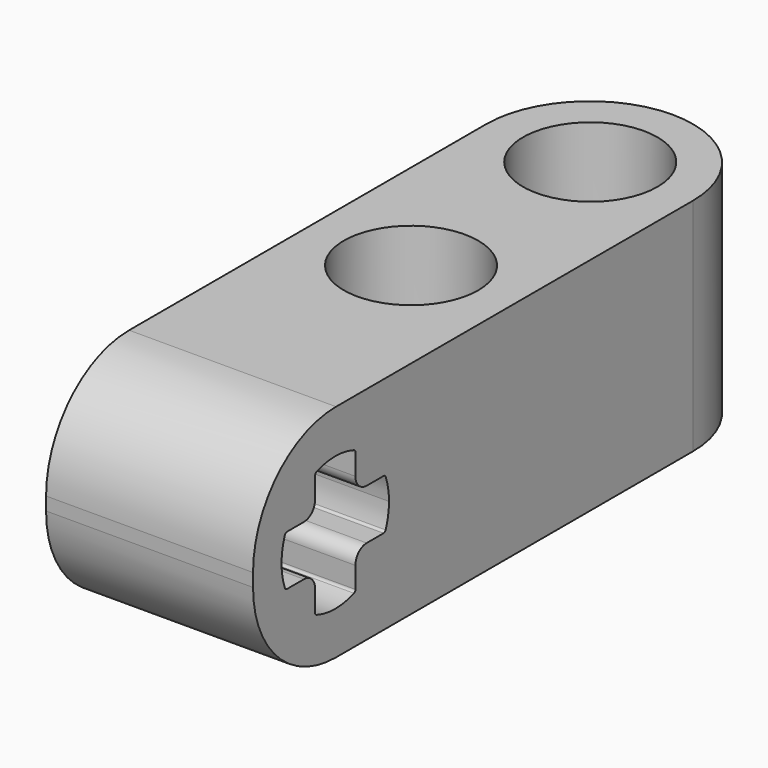
from build123d import *

# Parameters (mm, degrees)
F0_W        = 7.39
F0_H        = 23.34
F0_R        = 2.4
F1_DEPTH    = 7.88
F2_T1_DEPTH = 26.405
F4_DEPTH    = 7.391
F5_R        = 3.705


# Not quite as in the source:
# - a fillet or chamfer that OpenCascade refuses, or shapes differently, is made with other operations: its cross-section is extruded or revolved along the edge and cut away or added


with BuildPart() as f1:
    # F0 (on Top) → F1 (new body)
    with BuildSketch(Plane.XY):
        with Locations((-61.1013304442, -8.6294944299)):
            Rectangle(F0_W, F0_H)
        with Locations((-61.1013304442, -8.6294944299)):
            Circle(F0_R, mode=Mode.SUBTRACT)
        with Locations((-61.1013304442, -0.6294944299)):
            Circle(F0_R, mode=Mode.SUBTRACT)
    extrude(amount=F1_DEPTH)

    # F2: fillet of radius 3.705 on 2 edges, made by hand

    # F2_s2 → F2_t1 (cut)
    with BuildSketch(Plane.XY.offset(-9.2625)):
        with BuildLine():
            ThreePointArc((-61.0913304442, 3.0405055701), (-63.7111610685, 1.9553361944), (-64.7963304442, -0.6644944299))
            Line((-64.7963304442, -0.6644944299), (-64.7963304442, 3.0405055701))
            Line((-64.7963304442, 3.0405055701), (-61.0913304442, 3.0405055701))
        make_face()
        with BuildLine():
            ThreePointArc((-61.1113304442, 3.0405055701), (-58.4914998199, 1.9553361944), (-57.4063304442, -0.6644944299))
            Line((-57.4063304442, -0.6644944299), (-57.4063304442, 3.0405055701))
            Line((-57.4063304442, 3.0405055701), (-61.1113304442, 3.0405055701))
        make_face()
    extrude(amount=F2_T1_DEPTH, mode=Mode.SUBTRACT)

    # F3 (on face) → F4 (cut, through all)
    with BuildSketch(Plane.YZ.offset(-57.4063304442)):
        with BuildLine():
            Line((-15.7294944299, 5.34), (-15.7294944299, 6.0963858653))
            ThreePointArc((-15.7294944299, 6.0963858653), (-15.747402223, 6.1534898894), (-15.7947118212, 6.1901417725))
            ThreePointArc((-15.7947118212, 6.1901417725), (-16.6294944299, 6.34), (-17.4642770386, 6.1901417725))
            ThreePointArc((-17.4642770386, 6.1901417725), (-17.5115866368, 6.1534898894), (-17.5294944299, 6.0963858653))
            Line((-17.5294944299, 6.0963858653), (-17.5294944299, 5.34))
            ThreePointArc((-17.5294944299, 5.34), (-17.6759410393, 4.9864466094), (-18.0294944299, 4.84))
            Line((-18.0294944299, 4.84), (-18.7858802952, 4.84))
            ThreePointArc((-18.7858802952, 4.84), (-18.8429843193, 4.8220922069), (-18.8796362024, 4.7747826087))
            ThreePointArc((-18.8796362024, 4.7747826087), (-18.9917328021, 4.3640635248), (-19.0294944299, 3.94))
            ThreePointArc((-19.0294944299, 3.94), (-18.9917328021, 3.5159364752), (-18.8796362024, 3.1052173913))
            ThreePointArc((-18.8796362024, 3.1052173913), (-18.8429843193, 3.0579077931), (-18.7858802952, 3.04))
            Line((-18.7858802952, 3.04), (-18.0294944299, 3.04))
            ThreePointArc((-18.0294944299, 3.04), (-17.6759410393, 2.8935533906), (-17.5294944299, 2.54))
            Line((-17.5294944299, 2.54), (-17.5294944299, 1.7836141347))
            ThreePointArc((-17.5294944299, 1.7836141347), (-17.5115866368, 1.7265101106), (-17.4642770386, 1.6898582275))
            ThreePointArc((-17.4642770386, 1.6898582275), (-16.6294944299, 1.54), (-15.7947118212, 1.6898582275))
            ThreePointArc((-15.7947118212, 1.6898582275), (-15.747402223, 1.7265101106), (-15.7294944299, 1.7836141347))
            Line((-15.7294944299, 1.7836141347), (-15.7294944299, 2.54))
            ThreePointArc((-15.7294944299, 2.54), (-15.5830478205, 2.8935533906), (-15.2294944299, 3.04))
            Line((-15.2294944299, 3.04), (-14.4731085646, 3.04))
            ThreePointArc((-14.4731085646, 3.04), (-14.4160045405, 3.0579077931), (-14.3793526574, 3.1052173913))
            ThreePointArc((-14.3793526574, 3.1052173913), (-14.2672560577, 3.5159364752), (-14.2294944299, 3.94))
            ThreePointArc((-14.2294944299, 3.94), (-14.2672560577, 4.3640635248), (-14.3793526574, 4.7747826087))
            ThreePointArc((-14.3793526574, 4.7747826087), (-14.4160045405, 4.8220922069), (-14.4731085646, 4.84))
            Line((-14.4731085646, 4.84), (-15.2294944299, 4.84))
            ThreePointArc((-15.2294944299, 4.84), (-15.5830478205, 4.9864466094), (-15.7294944299, 5.34))
        make_face()
    extrude(amount=-F4_DEPTH, mode=Mode.SUBTRACT)

    # F5
    f5_edges = [f1.edges().sort_by_distance(p)[0] for p in [
        (-61.10133, -20.299494, 7.88),
        (-61.10133, -20.299494, 0),
    ]]
    fillet(f5_edges, radius=F5_R)


solid = f1.part
